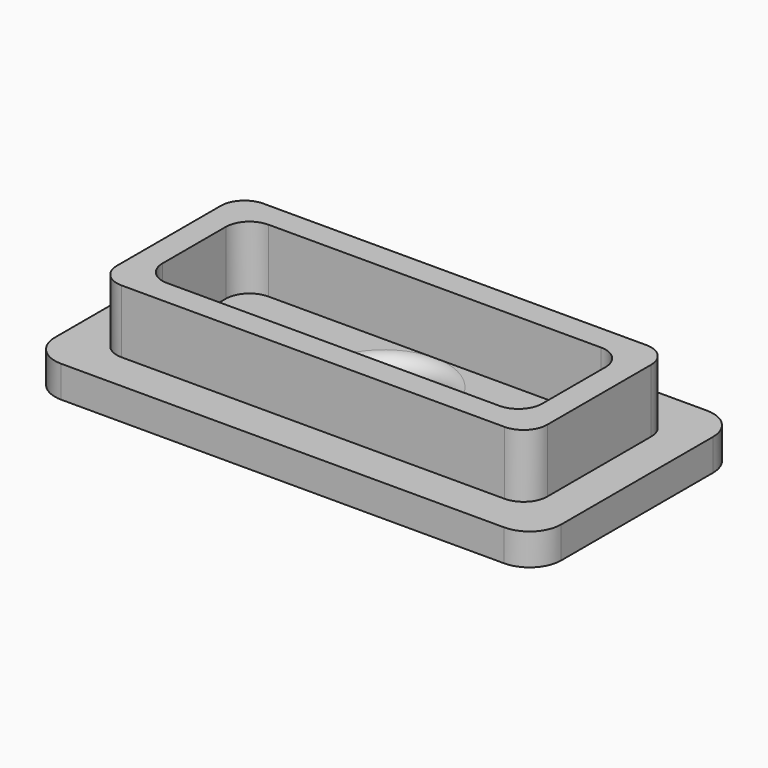
from build123d import *

# Parameters (mm, degrees)
F0_W     = 13.6
F0_H     = 5.6
F1_DEPTH = 3
F2_T     = -0.8
F3_W     = 16
F3_H     = 8
F4_DEPTH = 1
F5_R     = 0.75
F6_R     = 1
F7_R     = 1.5
F8_DEPTH = 25
F10_R    = 0.49999


# Not quite as in the source:
# - a fillet or chamfer is up to 0.001 mm smaller than in the source, because OpenCascade refuses the exact size


with BuildPart() as f1:
    # F0 (on Top) → F1 (new body)
    with BuildSketch(Plane.XY):
        Rectangle(F0_W, F0_H)
    extrude(amount=F1_DEPTH)

    # F2
    f2_openings = [f1.faces().sort_by_distance(p)[0] for p in [
        (0, 0, 3),
    ]]
    offset(amount=F2_T, openings=f2_openings)

    # F3 (on Top) → F4 (join)
    with BuildSketch(Plane.XY):
        Rectangle(F3_W, F3_H)
    extrude(amount=F4_DEPTH)

    # F5
    f5_edges = [f1.edges().sort_by_distance(p)[0] for p in [
        (6.8, -2.8, 2),
        (6.8, 2.8, 2),
        (6, 2, 2),
        (6, -2, 2),
        (-6, 2, 2),
        (-6, -2, 2),
        (-6.8, 2.8, 2),
        (-6.8, -2.8, 2),
    ]]
    fillet(f5_edges, radius=F5_R)

    # F6
    f6_edges = [f1.edges().sort_by_distance(p)[0] for p in [
        (-8, -4, 0.5),
        (8, -4, 0.5),
        (8, 4, 0.5),
        (-8, 4, 0.5),
    ]]
    fillet(f6_edges, radius=F6_R)


with BuildPart() as f8:
    # F7 (on Top) → F8 (new body)
    with BuildSketch(Plane.XY):
        Circle(F7_R)
    extrude(amount=F8_DEPTH)


with BuildPart() as f1_1:
    add(f1.part)

    # F9: cut F8
    add(f8.part, mode=Mode.SUBTRACT)

    # F10 (radius 0.5 in the source; OpenCascade refuses exactly that, so slightly less here)
    f10_edges = [f1_1.edges().sort_by_distance(p)[0] for p in [
        (-1.5, 0, 1),
    ]]
    fillet(f10_edges, radius=F10_R)


solid = f1_1.part
